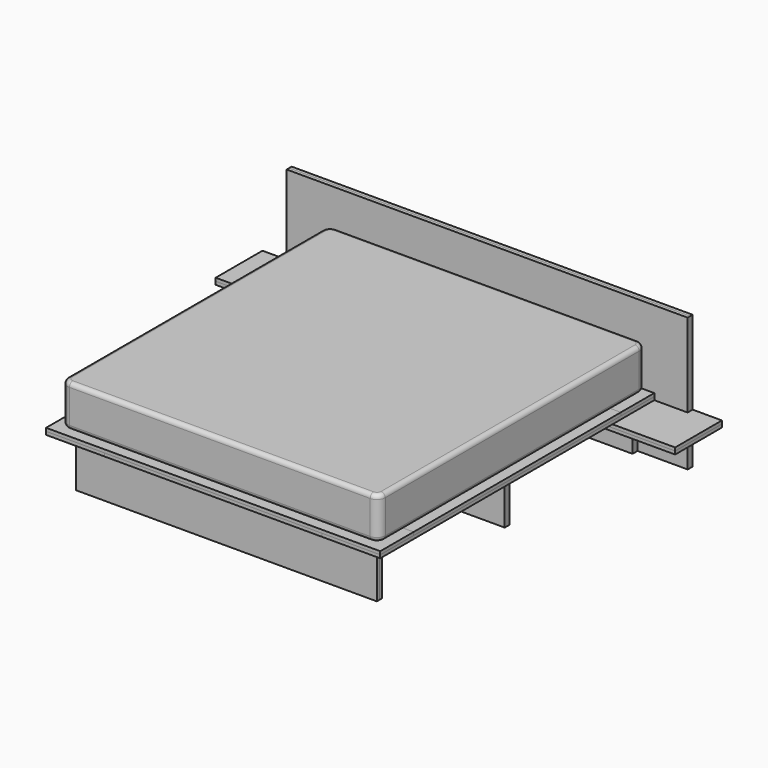
from build123d import *

# Parameters (mm, degrees)
F7_W      = 1219.2
F7_H      = 19.05
F8_DEPTH  = 812.8
F10_DEPTH = 812.8
F11_W     = 895.35
F11_H     = 19.05
F12_DEPTH = 304.8
F11_W_2   = 1828.8
F13_W     = 895.35
F13_H     = 19.05
F14_DEPTH = 304.8
F13_W_2   = 1828.8
F15_W     = 19.05
F15_H     = 1962.15
F16_DEPTH = 304.8
F17_W     = 19.05
F17_H     = 1962.15
F18_DEPTH = 304.8
F19_W     = 38.1
F19_H     = 152.4
F20_DEPTH = 1054.101
F21_W     = 38.1
F21_H     = 152.4000000002
F22_DEPTH = 76.2
F23_W     = 1320.8
F23_H     = 254
F24_DEPTH = 19.05
F25_W     = 355.6
F25_H     = 2082.8
F26_DEPTH = 19.05
F27_W     = 2032
F27_H     = 254
F28_DEPTH = 19.05
F29_W     = 254
F29_H     = 1574.8
F30_DEPTH = 19.05
F32_DEPTH = 19.05
F34_DEPTH = 19.05
F36_DEPTH = 254
F37_R     = 25.4


with BuildPart() as f8:
    # F7 (on Top) → F8 (new body)
    with BuildSketch(Plane.XY):
        with Locations((-609.6, 1025.525)):
            Rectangle(F7_W, F7_H)
        with Locations((609.6, 1025.525)):
            Rectangle(F7_W, F7_H)
    extrude(amount=F8_DEPTH)


with BuildPart() as f10:
    # F9 (on Top) → F10 (new body, through all)
    with BuildSketch(Plane.XY):
        Polygon((-1219.2, 1054.1), (-1219.2, 1035.05), (0, 1035.05), (1219.2, 1035.05), (1219.2, 1054.1), align=None)
    extrude(amount=F10_DEPTH)


with BuildPart() as f12:
    # F11 (on Top) → F12 (new body, through all)
    with BuildSketch(Plane.XY):
        with Locations((-466.725, 987.425)):
            Rectangle(F11_W, F11_H)
    extrude(amount=F12_DEPTH)


with BuildPart() as f12b:
    # F11 (on Top) → F12, piece 2 (new body, through all)
    with BuildSketch(Plane.XY):
        with Locations((466.725, 987.425)):
            Rectangle(F11_W, F11_H)
    extrude(amount=F12_DEPTH)


with BuildPart() as f12c:
    # F11 (on Top) → F12, piece 3 (new body, through all)
    with BuildSketch(Plane.XY):
        with Locations((0, 15.875)):
            Rectangle(F11_W_2, F11_H)
    extrude(amount=F12_DEPTH)


with BuildPart() as f12d:
    # F11 (on Top) → F12, piece 4 (new body, through all)
    with BuildSketch(Plane.XY):
        with Locations((0, -955.675)):
            Rectangle(F11_W_2, F11_H)
    extrude(amount=F12_DEPTH)


with BuildPart() as f14:
    # F13 (on Top) → F14 (new body, through all)
    with BuildSketch(Plane.XY):
        with Locations((-466.725, 1006.475)):
            Rectangle(F13_W, F13_H)
    extrude(amount=F14_DEPTH)


with BuildPart() as f14b:
    # F13 (on Top) → F14, piece 2 (new body, through all)
    with BuildSketch(Plane.XY):
        with Locations((466.725, 1006.475)):
            Rectangle(F13_W, F13_H)
    extrude(amount=F14_DEPTH)


with BuildPart() as f14c:
    # F13 (on Top) → F14, piece 3 (new body, through all)
    with BuildSketch(Plane.XY):
        with Locations((0, 34.925)):
            Rectangle(F13_W_2, F13_H)
    extrude(amount=F14_DEPTH)


with BuildPart() as f14d:
    # F13 (on Top) → F14, piece 4 (new body, through all)
    with BuildSketch(Plane.XY):
        with Locations((-466.725, -936.625)):
            Rectangle(F13_W, F13_H)
    extrude(amount=F14_DEPTH)


with BuildPart() as f14e:
    # F13 (on Top) → F14, piece 5 (new body, through all)
    with BuildSketch(Plane.XY):
        with Locations((466.725, -936.625)):
            Rectangle(F13_W, F13_H)
    extrude(amount=F14_DEPTH)


with BuildPart() as f16:
    # F15 (on Top) → F16 (new body, through all)
    with BuildSketch(Plane.XY):
        with Locations((-9.525, 34.925)):
            Rectangle(F15_W, F15_H)
    extrude(amount=F16_DEPTH)


with BuildPart() as f18:
    # F17 (on Top) → F18 (new body, through all)
    with BuildSketch(Plane.XY):
        with Locations((9.525, 34.925)):
            Rectangle(F17_W, F17_H)
    extrude(amount=F18_DEPTH)


with BuildPart() as f20_tool:
    # F19 (on Front) → F20 (new body, through all)
    with BuildSketch(Plane.XZ):
        with Locations((0, 228.6)):
            Rectangle(F19_W, F19_H)
    extrude(amount=-F20_DEPTH)


with BuildPart() as f12c_1:
    add(f12c.part)

    # F20: cut by f20_tool
    add(f20_tool.part, mode=Mode.SUBTRACT)


with BuildPart() as f14c_1:
    add(f14c.part)

    # F20: cut by f20_tool
    add(f20_tool.part, mode=Mode.SUBTRACT)


with BuildPart() as f22_tool:
    # F21 (on Right) → F22 (new body, symmetric)
    with BuildSketch(Plane.YZ):
        with Locations((25.4, 76.2000000001)):
            Rectangle(F21_W, F21_H)
    extrude(amount=F22_DEPTH, both=True)


with BuildPart() as f16_1:
    add(f16.part)

    # F22: cut by f22_tool
    add(f22_tool.part, mode=Mode.SUBTRACT)


with BuildPart() as f18_1:
    add(f18.part)

    # F22: cut by f22_tool
    add(f22_tool.part, mode=Mode.SUBTRACT)


with BuildPart() as f24:
    # F23 (on offset) → F24 (new body)
    with BuildSketch(Plane.XY.offset(304.8)):
        with Locations((0, 889)):
            Rectangle(F23_W, F23_H)
    extrude(amount=F24_DEPTH)


with BuildPart() as f24b:
    # F23 (on offset) → F24, piece 2 (new body)
    with BuildSketch(Plane.XY.offset(304.8)):
        with Locations((0, -939.8)):
            Rectangle(F23_W, F23_H)
    extrude(amount=F24_DEPTH)


with BuildPart() as f26:
    # F25 (on offset) → F26 (new body)
    with BuildSketch(Plane.XY.offset(304.8)):
        with Locations((-838.2, -25.4)):
            Rectangle(F25_W, F25_H)
    extrude(amount=F26_DEPTH)


with BuildPart() as f26b:
    # F25 (on offset) → F26, piece 2 (new body)
    with BuildSketch(Plane.XY.offset(304.8)):
        with Locations((838.2, -25.4)):
            Rectangle(F25_W, F25_H)
    extrude(amount=F26_DEPTH)


with BuildPart() as f28:
    # F27 (on face) → F28 (new body)
    with BuildSketch(Plane.XY.offset(323.85)):
        with Locations((0, 889)):
            Rectangle(F27_W, F27_H)
    extrude(amount=F28_DEPTH)


with BuildPart() as f28b:
    # F27 (on face) → F28, piece 2 (new body)
    with BuildSketch(Plane.XY.offset(323.85)):
        with Locations((0, -939.8)):
            Rectangle(F27_W, F27_H)
    extrude(amount=F28_DEPTH)


with BuildPart() as f30:
    # F29 (on face) → F30 (new body)
    with BuildSketch(Plane.XY.offset(323.85)):
        with Locations((-889, -25.4)):
            Rectangle(F29_W, F29_H)
    extrude(amount=F30_DEPTH)


with BuildPart() as f30b:
    # F29 (on face) → F30, piece 2 (new body)
    with BuildSketch(Plane.XY.offset(323.85)):
        with Locations((889, -25.4)):
            Rectangle(F29_W, F29_H)
    extrude(amount=F30_DEPTH)


with BuildPart() as f32:
    # F31 (on offset) → F32 (new body)
    with BuildSketch(Plane.XY.offset(304.8)):
        Polygon((-1397, 1054.1), (-1397, 698.5), (-762, 698.5), (-762, 977.9), (-914.4, 977.9), (-914.4, 1016), (-1219.2, 1016), (-1219.2, 1054.1), align=None)
    extrude(amount=-F32_DEPTH)


with BuildPart() as f32b:
    # F31 (on offset) → F32, piece 2 (new body)
    with BuildSketch(Plane.XY.offset(304.8)):
        Polygon((1397, 698.5), (1397, 1054.1), (1219.2, 1054.1), (1219.2, 1016), (914.4, 1016), (914.4, 977.9), (762, 977.9), (762, 698.5), align=None)
    extrude(amount=-F32_DEPTH)


with BuildPart() as f34:
    # F33 (on face) → F34 (new body)
    with BuildSketch(Plane(origin=(0, 0, 285.75), x_dir=(1, 0, 0), z_dir=(0, 0, -1))):
        Polygon((-762, -698.5), (-1397, -698.5), (-1397, -1054.1), (-1219.2, -1054.1), (-1219.2, -1016), (-914.4, -1016), (-914.4, -977.9), (-762, -977.9), align=None)
    extrude(amount=F34_DEPTH)


with BuildPart() as f34b:
    # F33 (on face) → F34, piece 2 (new body)
    with BuildSketch(Plane(origin=(0, 0, 285.75), x_dir=(1, 0, 0), z_dir=(0, 0, -1))):
        Polygon((1219.2, -1054.1), (1397, -1054.1), (1397, -698.5), (762, -698.5), (762, -977.9), (914.4, -977.9), (914.4, -1016), (1219.2, -1016), align=None)
    extrude(amount=F34_DEPTH)


with BuildPart() as f36:
    # F35 (on face) → F36 (new body)
    with BuildSketch(Plane.XY.offset(342.9)):
        with BuildLine():
            Line((0, 1016), (-914.4, 1016))
            ThreePointArc((-914.4, 1016), (-950.3210244843, 1001.1210244843), (-965.2, 965.2))
            Line((-965.2, 965.2), (-965.2, -965.2))
            ThreePointArc((-965.2, -965.2), (-950.3210244843, -1001.1210244843), (-914.4, -1016))
            Line((-914.4, -1016), (0, -1016))
            Line((0, -1016), (0, 1016))
        make_face()
        with BuildLine():
            Line((914.4, 1016), (0, 1016))
            Line((0, 1016), (0, -1016))
            Line((0, -1016), (914.4, -1016))
            ThreePointArc((914.4, -1016), (950.3210244843, -1001.1210244843), (965.2, -965.2))
            Line((965.2, -965.2), (965.2, 965.2))
            ThreePointArc((965.2, 965.2), (950.3210244843, 1001.1210244843), (914.4, 1016))
        make_face()
    extrude(amount=F36_DEPTH)

    # F37
    f37_edges = [f36.edges().sort_by_distance(p)[0] for p in [
        (0, -1016, 596.9),
        (0, -1016, 342.9),
        (-950.321024, 1001.121024, 596.9),
        (-965.2, 0, 596.9),
        (-950.321024, -1001.121024, 596.9),
        (950.321024, -1001.121024, 596.9),
        (965.2, 0, 596.9),
        (950.321024, 1001.121024, 596.9),
    ]]
    fillet(f37_edges, radius=F37_R)


solid = Compound([f8.part, f10.part, f12.part, f12b.part, f12d.part, f14.part, f14b.part, f14d.part, f14e.part, f12c_1.part, f14c_1.part, f16_1.part, f18_1.part, f24.part, f24b.part, f26.part, f26b.part, f28.part, f28b.part, f30.part, f30b.part, f32.part, f32b.part, f34.part, f34b.part, f36.part])
